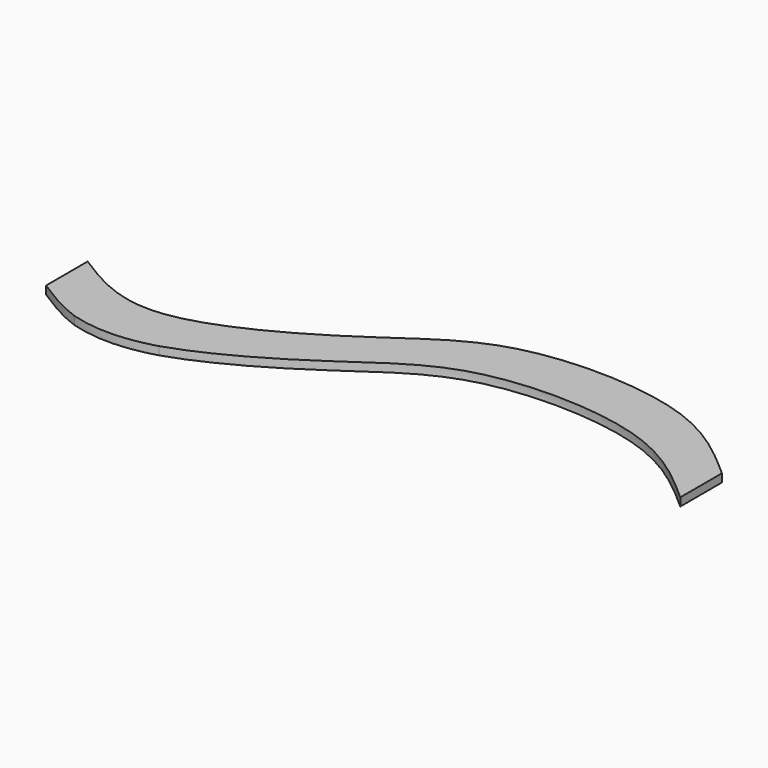
from build123d import *

# Parameters (mm, degrees)
F1_DEPTH = 0.6


# Not quite as in the source:
# - ends of sketch curves that miss each other by under 0.0002 mm in the source are joined


with BuildPart() as f1:
    # F0 (on Top) → F1 (new body)
    with BuildSketch(Plane.XY):
        with BuildLine():
            add(Edge.make_bspline(
                [(-27.683602202, 4.3622240029), (-25.358796936, 2.84664598), (-20.5608734618, 0.2826177406), (-8.9542219297, 6.8655938987), (-2.3967650886, 12.3788446821), (11.1135658845, 12.0190665422), (15.3822705643, 8.2562465754), (17.316397798, 6.5484584641)],
                knots=[0, 0, 0, 0, 0.1765674616, 0.400525264, 0.5930940384, 0.8177624668, 1, 1, 1, 1], degree=3))
            Line((-27.683602202, 4.3622240029), (-27.683602202, 0.5283586101))
            add(Edge.make_bspline(
                [(-27.683602202, 0.5283586101), (-26.4505713043, -0.2754743949), (-25.2765264365, -0.9709345602), (-24.0420313354, -1.4122566)],
                knots=[0, 0, 0, 0, 0.0936479357, 0.0936479357, 0.0936479357, 0.0936479357], degree=3))
            add(Edge.make_bspline(
                [(-24.0420313354, -1.4122566), (-22.7413190859, -1.7919411675), (-20.7616668205, -1.9846677675), (-18.5750781824, -1.5127811233), (-17.8813856832, -1.3136689309)],
                knots=[0.0896789193, 0.0896789193, 0.0896789193, 0.0896789193, 0.182373931, 0.2245564082, 0.2245564082, 0.2245564082, 0.2245564082], degree=3))
            add(Edge.make_bspline(
                [(-17.8813856832, -1.3136689309), (-15.0305462556, -0.3944745735), (-8.3944877894, 3.5023312426), (-2.3967655326, 8.5449792893), (11.1135654405, 8.1852011494), (15.3822701203, 4.4223811826), (17.316397354, 2.7145930713)],
                knots=[0.2312988961, 0.2312988961, 0.2312988961, 0.2312988961, 0.400525264, 0.5930940384, 0.8177624668, 1, 1, 1, 1], degree=3))
            Line((17.316397354, 2.7145930713), (17.316397798, 6.5484584641))
        make_face()
    extrude(amount=F1_DEPTH)


solid = f1.part
